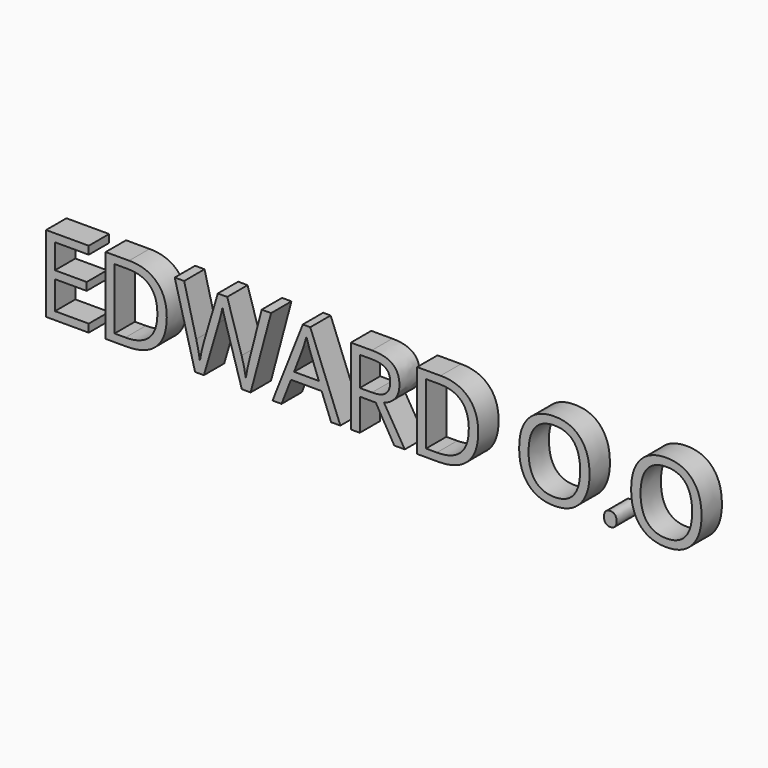
from build123d import *

# Parameters (mm, degrees)
F0_TEXT_SIZE = 213.7828721768
F1_DEPTH     = 50.8


# Not quite as in the source:
# - Text() gives the source's letters only with a copy of the font that has no kerning and outlines rounded to 1/6400 em; it was checked with that copy


with BuildPart() as f1:
    # F0 (on Front) → F1 (new body)
    with BuildSketch(Plane.XZ):
        with Locations((-127.650976181, -79.1036263108)):
            Text('EDWARD O.O', F0_TEXT_SIZE, font='Open Sans', text_align=(TextAlign.LEFT, TextAlign.BOTTOM))
    extrude(amount=F1_DEPTH)


solid = f1.part
